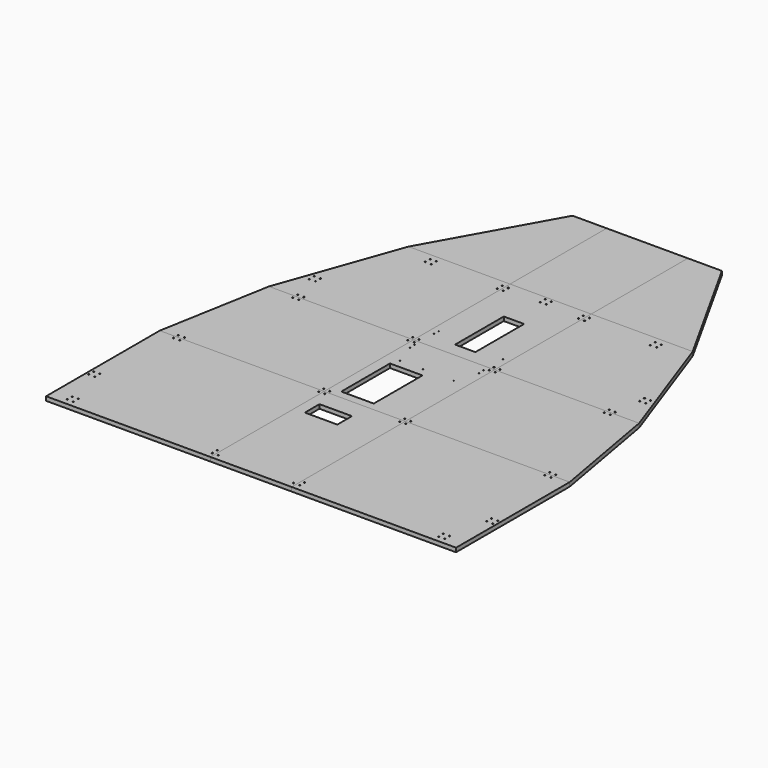
from build123d import *

# Parameters (mm, degrees)
F0_W      = 400
F0_H      = 700
F0_R      = 3
F0_W_2    = 160
F0_H_2    = 89.9538263201
F1_DEPTH  = 20
F2_R      = 3
F3_DEPTH  = 20
F4_DEPTH  = 20
F5_W      = 400
F5_H      = 550
F5_R      = 3
F5_W_2    = 160
F5_H_2    = 300
F5_R_2    = 2.05
F6_DEPTH  = 20
F7_W      = 400
F7_H      = 595
F7_R      = 3
F7_R_2    = 2.05
F7_W_2    = 100
F7_H_2    = 300
F8_DEPTH  = 20
F9_W      = 760
F9_H      = 700
F9_R      = 3
F10_DEPTH = 20
F11_W     = 400
F11_H     = 595
F12_DEPTH = 20
F14_DEPTH = 20
F16_DEPTH = 20
F17_W     = 50
F17_H     = 700
F17_R     = 3
F19_DEPTH = 20
F18_W     = 50
F18_H     = 700
F18_R     = 3
F20_DEPTH = 20
F21_R     = 3
F23_DEPTH = 20
F22_R     = 3
F24_DEPTH = 20
F26_DEPTH = 20
F28_DEPTH = 20
F30_DEPTH = 20
F32_DEPTH = 20


with BuildPart() as f1:
    # F0 (on Top) → F1 (new body)
    with BuildSketch(Plane.XY):
        Rectangle(F0_W, F0_H)
        with Locations((-185, -320)):
            Circle(F0_R, mode=Mode.SUBTRACT)
        with Locations((185, -320)):
            Circle(F0_R, mode=Mode.SUBTRACT)
        with Locations((-185, 335)):
            Circle(F0_R, mode=Mode.SUBTRACT)
        with Locations((-67.5, 210.6490433216)):
            Rectangle(F0_W_2, F0_H_2, mode=Mode.SUBTRACT)
        with Locations((185, 335)):
            Circle(F0_R, mode=Mode.SUBTRACT)
    extrude(amount=F1_DEPTH)


with BuildPart() as f3:
    # F2 (on Top) → F3 (new body)
    with BuildSketch(Plane.XY):
        Polygon((-200, 350), (-200, 900), (-812, 900), (-960, 350), align=None)
        with Locations((-930, 365)):
            Circle(F2_R, mode=Mode.SUBTRACT)
        with Locations((-900, 365)):
            Circle(F2_R, mode=Mode.SUBTRACT)
        with Locations((-215, 365)):
            Circle(F2_R, mode=Mode.SUBTRACT)
        with Locations((-782, 885)):
            Circle(F2_R, mode=Mode.SUBTRACT)
        with Locations((-752, 885)):
            Circle(F2_R, mode=Mode.SUBTRACT)
        with Locations((-215, 885)):
            Circle(F2_R, mode=Mode.SUBTRACT)
    extrude(amount=F3_DEPTH)

    # F25 (on face) → F26 (join)
    with BuildSketch(Plane(origin=(0, 0, 0), x_dir=(1, 0, 0), z_dir=(0, 0, -1))):
        Polygon((-912, -900), (-812, -900), (-960, -350), (-1010, -350), align=None)
    extrude(amount=-F26_DEPTH)


with BuildPart() as f3b:
    # F2 (on Top) → F3, piece 2 (new body)
    with BuildSketch(Plane.XY):
        Polygon((812, 900), (200, 900), (200, 350), (960, 350), align=None)
        with Locations((215, 365)):
            Circle(F2_R, mode=Mode.SUBTRACT)
        with Locations((900, 365)):
            Circle(F2_R, mode=Mode.SUBTRACT)
        with Locations((930, 365)):
            Circle(F2_R, mode=Mode.SUBTRACT)
        with Locations((215, 885)):
            Circle(F2_R, mode=Mode.SUBTRACT)
        with Locations((752, 885)):
            Circle(F2_R, mode=Mode.SUBTRACT)
        with Locations((782, 885)):
            Circle(F2_R, mode=Mode.SUBTRACT)
    extrude(amount=F3_DEPTH)

    # F27 (on face) → F28 (join)
    with BuildSketch(Plane(origin=(0, 0, 0), x_dir=(1, 0, 0), z_dir=(0, 0, -1))):
        Polygon((1010, -350), (960, -350), (812, -900), (912, -900), align=None)
    extrude(amount=-F28_DEPTH)


with BuildPart() as f4:
    # F2 (on Top) → F4 (new body)
    with BuildSketch(Plane.XY):
        Polygon((-812, 900), (-200, 900), (-200, 1495), (-600, 1495), align=None)
        with Locations((-782, 915)):
            Circle(F2_R, mode=Mode.SUBTRACT)
        with Locations((-752, 915)):
            Circle(F2_R, mode=Mode.SUBTRACT)
        with Locations((-215, 915)):
            Circle(F2_R, mode=Mode.SUBTRACT)
        with Locations((-570, 1435)):
            Circle(F2_R, mode=Mode.SUBTRACT)
        with Locations((-540, 1435)):
            Circle(F2_R, mode=Mode.SUBTRACT)
        with Locations((-570, 1465)):
            Circle(F2_R, mode=Mode.SUBTRACT)
        with Locations((-540, 1465)):
            Circle(F2_R, mode=Mode.SUBTRACT)
        with Locations((-215, 1435)):
            Circle(F2_R, mode=Mode.SUBTRACT)
        with Locations((-215, 1465)):
            Circle(F2_R, mode=Mode.SUBTRACT)
    extrude(amount=F4_DEPTH)

    # F21 (on face) → F23 (join)
    with BuildSketch(Plane(origin=(0, 0, 0), x_dir=(1, 0, 0), z_dir=(0, 0, -1))):
        Polygon((-700, -1495), (-600, -1495), (-812, -900), (-912, -900), align=None)
        with Locations((-828.5, -1075)):
            Circle(F21_R, mode=Mode.SUBTRACT)
        with Locations((-798.5, -1075)):
            Circle(F21_R, mode=Mode.SUBTRACT)
        with Locations((-828.5, -1045)):
            Circle(F21_R, mode=Mode.SUBTRACT)
        with Locations((-798.5, -1045)):
            Circle(F21_R, mode=Mode.SUBTRACT)
    extrude(amount=-F23_DEPTH)


with BuildPart() as f4b:
    # F2 (on Top) → F4, piece 2 (new body)
    with BuildSketch(Plane.XY):
        Polygon((600, 1495), (200, 1495), (200, 900), (812, 900), align=None)
        with Locations((215, 915)):
            Circle(F2_R, mode=Mode.SUBTRACT)
        with Locations((752, 915)):
            Circle(F2_R, mode=Mode.SUBTRACT)
        with Locations((782, 915)):
            Circle(F2_R, mode=Mode.SUBTRACT)
        with Locations((215, 1435)):
            Circle(F2_R, mode=Mode.SUBTRACT)
        with Locations((215, 1465)):
            Circle(F2_R, mode=Mode.SUBTRACT)
        with Locations((540, 1435)):
            Circle(F2_R, mode=Mode.SUBTRACT)
        with Locations((570, 1435)):
            Circle(F2_R, mode=Mode.SUBTRACT)
        with Locations((540, 1465)):
            Circle(F2_R, mode=Mode.SUBTRACT)
        with Locations((570, 1465)):
            Circle(F2_R, mode=Mode.SUBTRACT)
    extrude(amount=F4_DEPTH)

    # F22 (on face) → F24 (join)
    with BuildSketch(Plane(origin=(0, 0, 0), x_dir=(1, 0, 0), z_dir=(0, 0, -1))):
        Polygon((912, -900), (812, -900), (600, -1495), (700, -1495), align=None)
        with Locations((798.415464569, -1075)):
            Circle(F22_R, mode=Mode.SUBTRACT)
        with Locations((828.415464569, -1075)):
            Circle(F22_R, mode=Mode.SUBTRACT)
        with Locations((798.415464569, -1045)):
            Circle(F22_R, mode=Mode.SUBTRACT)
        with Locations((828.415464569, -1045)):
            Circle(F22_R, mode=Mode.SUBTRACT)
    extrude(amount=-F24_DEPTH)


with BuildPart() as f6:
    # F5 (on Top) → F6 (new body)
    with BuildSketch(Plane.XY):
        with Locations((0, 625)):
            Rectangle(F5_W, F5_H)
        with Locations((-185, 365)):
            Circle(F5_R, mode=Mode.SUBTRACT)
        with Locations((-67.5, 540)):
            Rectangle(F5_W_2, F5_H_2, mode=Mode.SUBTRACT)
        with Locations((185, 365)):
            Circle(F5_R, mode=Mode.SUBTRACT)
        with Locations((-132.5, 731.5)):
            Circle(F5_R_2, mode=Mode.SUBTRACT)
        with Locations((-17.5, 731.5)):
            Circle(F5_R_2, mode=Mode.SUBTRACT)
        with Locations((-170, 840)):
            Circle(F5_R_2, mode=Mode.SUBTRACT)
        with Locations((-185, 885)):
            Circle(F5_R, mode=Mode.SUBTRACT)
        with Locations((-170, 870)):
            Circle(F5_R_2, mode=Mode.SUBTRACT)
        with Locations((132.5, 731.5)):
            Circle(F5_R_2, mode=Mode.SUBTRACT)
        with Locations((170, 840)):
            Circle(F5_R_2, mode=Mode.SUBTRACT)
        with Locations((170, 870)):
            Circle(F5_R_2, mode=Mode.SUBTRACT)
        with Locations((185, 885)):
            Circle(F5_R, mode=Mode.SUBTRACT)
    extrude(amount=F6_DEPTH)


with BuildPart() as f8:
    # F7 (on Top) → F8 (new body)
    with BuildSketch(Plane.XY):
        with Locations((0, 1197.5)):
            Rectangle(F7_W, F7_H)
        with Locations((-185, 915)):
            Circle(F7_R, mode=Mode.SUBTRACT)
        with Locations((-170, 988)):
            Circle(F7_R_2, mode=Mode.SUBTRACT)
        with Locations((-170, 1018)):
            Circle(F7_R_2, mode=Mode.SUBTRACT)
        with Locations((185, 915)):
            Circle(F7_R, mode=Mode.SUBTRACT)
        with Locations((170, 988)):
            Circle(F7_R_2, mode=Mode.SUBTRACT)
        with Locations((170, 1018)):
            Circle(F7_R_2, mode=Mode.SUBTRACT)
        with Locations((0, 1119.0668344498)):
            Rectangle(F7_W_2, F7_H_2, mode=Mode.SUBTRACT)
        with Locations((-185, 1435)):
            Circle(F7_R, mode=Mode.SUBTRACT)
        with Locations((-185, 1465)):
            Circle(F7_R, mode=Mode.SUBTRACT)
        with Locations((-15, 1450)):
            Circle(F7_R, mode=Mode.SUBTRACT)
        with Locations((-15, 1480)):
            Circle(F7_R, mode=Mode.SUBTRACT)
        with Locations((15, 1450)):
            Circle(F7_R, mode=Mode.SUBTRACT)
        with Locations((15, 1480)):
            Circle(F7_R, mode=Mode.SUBTRACT)
        with Locations((185, 1435)):
            Circle(F7_R, mode=Mode.SUBTRACT)
        with Locations((185, 1465)):
            Circle(F7_R, mode=Mode.SUBTRACT)
    extrude(amount=F8_DEPTH)


with BuildPart() as f10:
    # F9 (on Top) → F10 (new body)
    with BuildSketch(Plane.XY):
        with Locations((-580, 0)):
            Rectangle(F9_W, F9_H)
        with Locations((-930, -320)):
            Circle(F9_R, mode=Mode.SUBTRACT)
        with Locations((-900, -320)):
            Circle(F9_R, mode=Mode.SUBTRACT)
        with Locations((-930, -290)):
            Circle(F9_R, mode=Mode.SUBTRACT)
        with Locations((-900, -290)):
            Circle(F9_R, mode=Mode.SUBTRACT)
        with Locations((-215, -320)):
            Circle(F9_R, mode=Mode.SUBTRACT)
        with Locations((-215, -290)):
            Circle(F9_R, mode=Mode.SUBTRACT)
        with Locations((-930, 335)):
            Circle(F9_R, mode=Mode.SUBTRACT)
        with Locations((-900, 335)):
            Circle(F9_R, mode=Mode.SUBTRACT)
        with Locations((-215, 335)):
            Circle(F9_R, mode=Mode.SUBTRACT)
    extrude(amount=F10_DEPTH)

    # F17 (on face) → F19 (join)
    with BuildSketch(Plane(origin=(0, 0, 0), x_dir=(1, 0, 0), z_dir=(0, 0, -1))):
        with Locations((-985, 0)):
            Rectangle(F17_W, F17_H)
        with Locations((-995, 75)):
            Circle(F17_R, mode=Mode.SUBTRACT)
        with Locations((-995, 105)):
            Circle(F17_R, mode=Mode.SUBTRACT)
        with Locations((-965, 75)):
            Circle(F17_R, mode=Mode.SUBTRACT)
        with Locations((-965, 105)):
            Circle(F17_R, mode=Mode.SUBTRACT)
    extrude(amount=-F19_DEPTH)


with BuildPart() as f10b:
    # F9 (on Top) → F10, piece 2 (new body)
    with BuildSketch(Plane.XY):
        with Locations((580, 0)):
            Rectangle(F9_W, F9_H)
        with Locations((215, -320)):
            Circle(F9_R, mode=Mode.SUBTRACT)
        with Locations((215, -290)):
            Circle(F9_R, mode=Mode.SUBTRACT)
        with Locations((900, -320)):
            Circle(F9_R, mode=Mode.SUBTRACT)
        with Locations((930, -320)):
            Circle(F9_R, mode=Mode.SUBTRACT)
        with Locations((900, -290)):
            Circle(F9_R, mode=Mode.SUBTRACT)
        with Locations((930, -290)):
            Circle(F9_R, mode=Mode.SUBTRACT)
        with Locations((215, 335)):
            Circle(F9_R, mode=Mode.SUBTRACT)
        with Locations((900, 335)):
            Circle(F9_R, mode=Mode.SUBTRACT)
        with Locations((930, 335)):
            Circle(F9_R, mode=Mode.SUBTRACT)
    extrude(amount=F10_DEPTH)

    # F18 (on face) → F20 (join)
    with BuildSketch(Plane(origin=(0, 0, 0), x_dir=(1, 0, 0), z_dir=(0, 0, -1))):
        with Locations((985, 0)):
            Rectangle(F18_W, F18_H)
        with Locations((965, 75)):
            Circle(F18_R, mode=Mode.SUBTRACT)
        with Locations((965, 105)):
            Circle(F18_R, mode=Mode.SUBTRACT)
        with Locations((995, 75)):
            Circle(F18_R, mode=Mode.SUBTRACT)
        with Locations((995, 105)):
            Circle(F18_R, mode=Mode.SUBTRACT)
    extrude(amount=-F20_DEPTH)


with BuildPart() as f12:
    # F11 (on face) → F12 (new body)
    with BuildSketch(Plane.XY.offset(20)):
        with Locations((0, 1792.5)):
            Rectangle(F11_W, F11_H)
    extrude(amount=-F12_DEPTH)


with BuildPart() as f14:
    # F13 (on face) → F14 (new body)
    with BuildSketch(Plane.XY.offset(20)):
        Polygon((-600, 1495), (-200, 1495), (-200, 2090), (-268, 2090), align=None)
    extrude(amount=-F14_DEPTH)

    # F31 (on face) → F32 (join)
    with BuildSketch(Plane(origin=(0, 0, 0), x_dir=(1, 0, 0), z_dir=(0, 0, -1))):
        Polygon((-268, -2090), (-600, -1495), (-700, -1495), (-368, -2090), align=None)
    extrude(amount=-F32_DEPTH)


with BuildPart() as f16:
    # F15 (on face) → F16 (new body)
    with BuildSketch(Plane.XY.offset(20)):
        Polygon((200, 2090), (200, 1495), (600, 1495), (268, 2090), align=None)
    extrude(amount=-F16_DEPTH)

    # F29 (on face) → F30 (join)
    with BuildSketch(Plane(origin=(0, 0, 0), x_dir=(1, 0, 0), z_dir=(0, 0, -1))):
        Polygon((700, -1495), (600, -1495), (268, -2090), (368, -2090), align=None)
    extrude(amount=-F30_DEPTH)


solid = Compound([f1.part, f3.part, f3b.part, f4.part, f4b.part, f6.part, f8.part, f10.part, f10b.part, f12.part, f14.part, f16.part])
